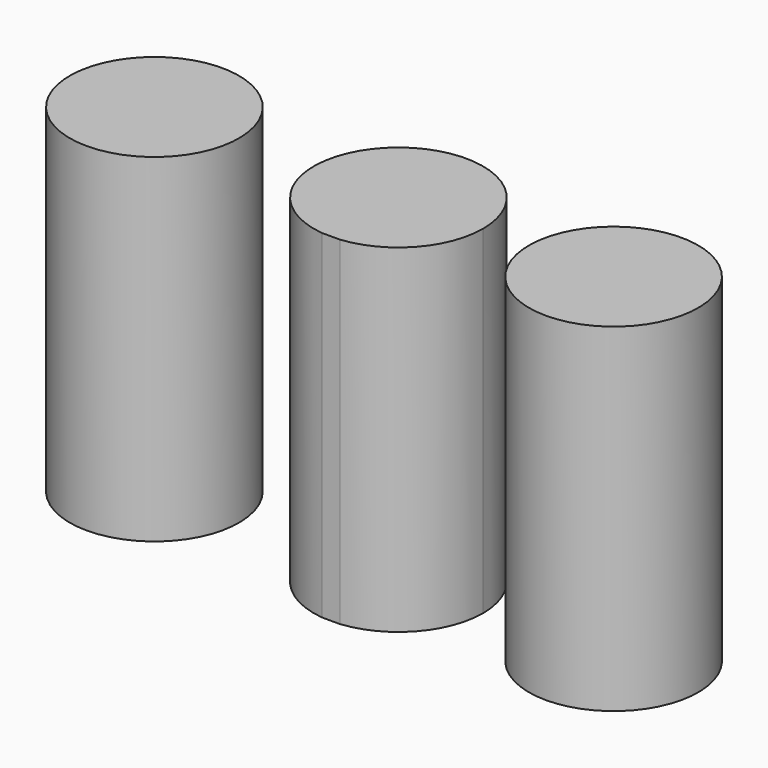
from build123d import *

# Parameters (mm, degrees)
F1_DEPTH = 30


# Not quite as in the source:
# - the program builds the solid bodies; features that only make, move or delete a surface that nothing else refers to are left out


with BuildPart() as f1:
    # F0 (on Top) → F1 (new body)
    with BuildSketch(Plane.XY):
        with BuildLine():
            ThreePointArc((26.8999968469, 0), (24.7032977058, 5.3033008589), (19.3999968469, 7.5))
            ThreePointArc((19.3999968469, 7.5), (11.8999968469, 0), (19.3999968469, -7.5))
            ThreePointArc((19.3999968469, -7.5), (24.7032977058, -5.3033008589), (26.8999968469, 0))
        make_face()
    extrude(amount=F1_DEPTH)


with BuildPart() as f1b:
    # F0 (on Top) → F1, piece 2 (new body)
    with BuildSketch(Plane.XY):
        with BuildLine():
            ThreePointArc((-13.8000029325, 0), (-15.9967020736, 5.3033008589), (-21.3000029325, 7.5))
            ThreePointArc((-21.3000029325, 7.5), (-28.8000029325, 0), (-21.3000029325, -7.5))
            ThreePointArc((-21.3000029325, -7.5), (-15.9967020736, -5.3033008589), (-13.8000029325, 0))
        make_face()
    extrude(amount=F1_DEPTH)


with BuildPart() as f1c:
    # F0 (on Top) → F1, piece 3 (new body)
    with BuildSketch(Plane.XY):
        with BuildLine():
            Line((-0.4291974003, -7.5), (1.1508829887, -7.5))
            ThreePointArc((1.1508829887, -7.5), (5.9364728688, -5.0579356316), (7.8608427942, -0.0417269766))
            ThreePointArc((7.8608427942, -0.0417269766), (-4.6553658608, 5.533903098), (-0.4291974003, -7.5))
        make_face()
    extrude(amount=F1_DEPTH)


solid = Compound([f1.part, f1b.part, f1c.part])
